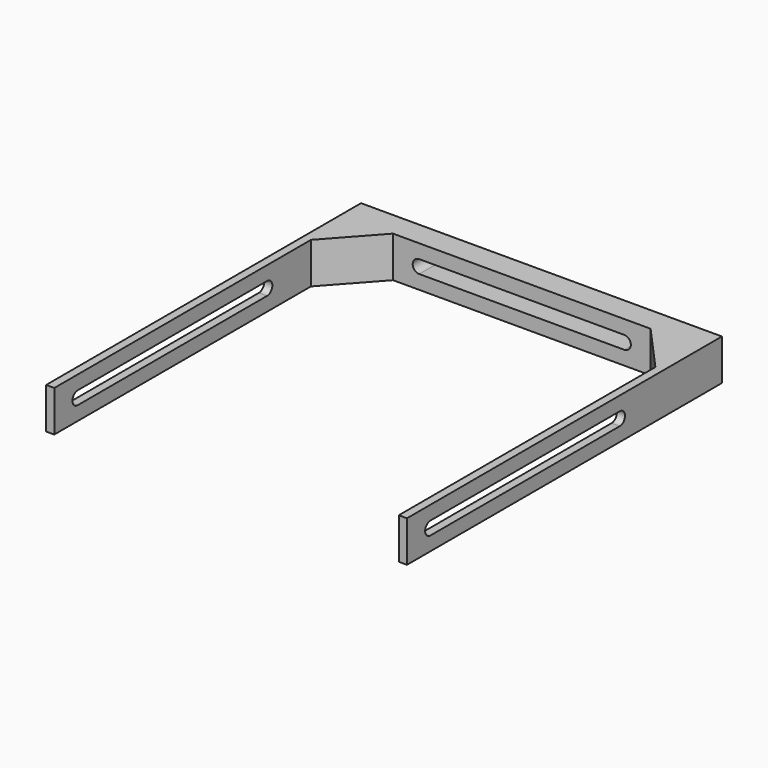
from build123d import *

# Parameters (mm, degrees)
F0_W     = 220
F0_H     = 25
F1_DEPTH = 15
F2_W     = 5
F2_H     = 25
F3_DEPTH = 225
F5_DEPTH = 25
F6_W     = 72.1634626389
F6_H     = 8
F7_DEPTH = 256


with BuildPart() as f1:
    # F0 (on Front) → F1 (new body)
    with BuildSketch(Plane.XZ):
        Rectangle(F0_W, F0_H)
        with BuildLine():
            Line((-62.5, 4), (62.5, 4))
            ThreePointArc((62.5, 4), (66.5, 0), (62.5, -4))
            Line((62.5, -4), (-62.5, -4))
            ThreePointArc((-62.5, -4), (-66.5, 0), (-62.5, 4))
        make_face(mode=Mode.SUBTRACT)
    extrude(amount=F1_DEPTH)

    # F2 (on face) → F3 (join)
    with BuildSketch(Plane.XZ.offset(15)):
        with Locations((-107.5, 0)):
            Rectangle(F2_W, F2_H)
        with Locations((107.5, 0)):
            Rectangle(F2_W, F2_H)
    extrude(amount=F3_DEPTH)

    # F4 (on face) → F5 (join)
    with BuildSketch(Plane(origin=(0, 0, -12.5), x_dir=(1, 0, 0), z_dir=(0, 0, -1))):
        Polygon((-110, 0), (-65, 0), (-110, 50), align=None)
        Polygon((65, 0), (110, 0), (110, 50), align=None)
    extrude(amount=-F5_DEPTH)

    # F6 (on face) → F7 (cut)
    with BuildSketch(Plane(origin=(-110, 0, 0), x_dir=(0, -1, 0), z_dir=(-1, 0, 0))):
        with Locations((186.076104641, 0)):
            Rectangle(F6_W, F6_H)
        with Locations((113.9126420021, 0)):
            Rectangle(F6_W, F6_H)
        with BuildLine():
            ThreePointArc((222.1578359604, -4), (226.1578359604, 0), (222.1578359604, 4))
            Line((222.1578359604, 4), (222.1578359604, -4))
        make_face()
        with BuildLine():
            Line((77.8309106827, -4), (77.8309106827, 4))
            ThreePointArc((77.8309106827, 4), (73.8309106827, 0), (77.8309106827, -4))
        make_face()
    extrude(amount=-F7_DEPTH, mode=Mode.SUBTRACT)


solid = f1.part
